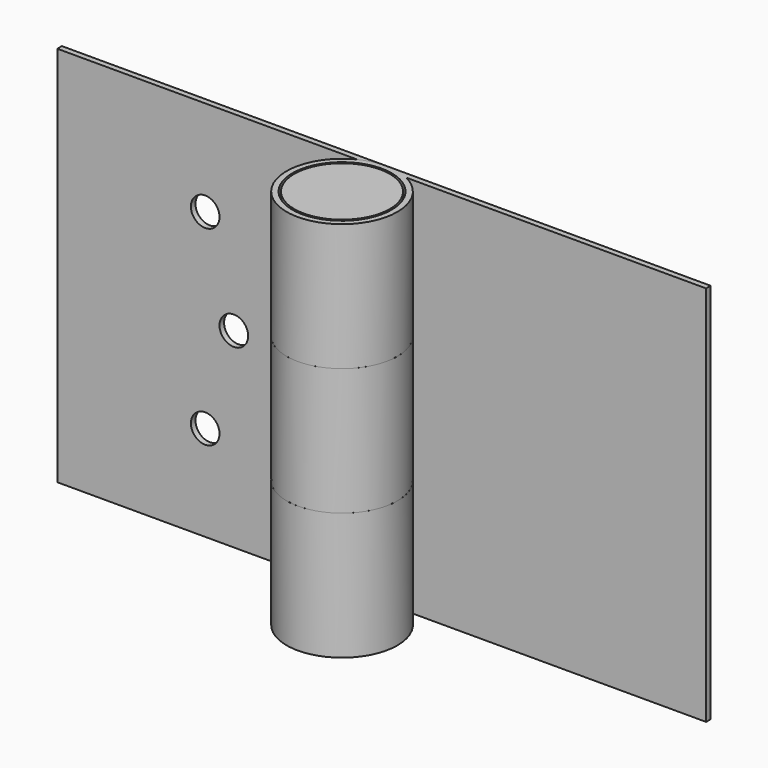
from build123d import *

# Parameters (mm, degrees)
F1_W      = 25
F1_H      = 200
F3_R      = 29
F3_R_2    = 26
F4_DEPTH  = 66.6666666667
F5_START  = -133.332
F5_DEPTH  = 66.668
F6_START  = -66.6666666667
F6_DEPTH  = 66.6666666667
F7_W      = 170
F7_H      = 3
F8_DEPTH  = 200
F9_W      = 170
F9_H      = 3
F10_DEPTH = 200
F11_R     = 7.5
F12_DEPTH = 25


with BuildPart() as f2:
    # F1 (on Front) → F2 (revolve)
    with BuildSketch(Plane.XZ):
        with Locations((-12.5, 0)):
            Rectangle(F1_W, F1_H)
    revolve(axis=Axis((0, 0, 0), (0, 0, -1)))


with BuildPart() as f4:
    # F3 (on face) → F4 (new body)
    with BuildSketch(Plane.XY.offset(100)):
        Circle(F3_R)
        Circle(F3_R_2, mode=Mode.SUBTRACT)
    extrude(amount=-F4_DEPTH)



with BuildPart() as f5:
    # F3 (on face) → F5 (new body)
    with BuildSketch(Plane.XY.offset(100).offset(F5_START)):
        Circle(F3_R)
        Circle(F3_R_2, mode=Mode.SUBTRACT)
    extrude(amount=-F5_DEPTH)


with BuildPart() as f6:
    # F3 (on face) → F6 (new body)
    with BuildSketch(Plane.XY.offset(100).offset(F6_START)):
        Circle(F3_R)
        Circle(F3_R_2, mode=Mode.SUBTRACT)
    extrude(amount=-F6_DEPTH)

    # F9 (on face) → F10 (join)
    with BuildSketch(Plane.XY.offset(100)):
        with Locations((-85, 27.5)):
            Rectangle(F9_W, F9_H)
    extrude(amount=-F10_DEPTH)

    # F11 (on face) → F12 (cut)
    with BuildSketch(Plane(origin=(0, 29, 0), x_dir=(-1, 0, 0), z_dir=(0, 1, 0))):
        with Locations((77.5, 0)):
            Circle(F11_R)
        with Locations((92.5, 50)):
            Circle(F11_R)
        with Locations((92.5, -50)):
            Circle(F11_R)
    extrude(amount=-F12_DEPTH, mode=Mode.SUBTRACT)


with BuildPart() as f4_1:
    add(f4.part)

    add(f5.part)  # F8 merges F5
    # F7 (on face) → F8 (join)
    with BuildSketch(Plane.XY.offset(100)):
        with Locations((85, 27.5)):
            Rectangle(F7_W, F7_H)
    extrude(amount=-F8_DEPTH)


solid = Compound([f2.part, f6.part, f4_1.part])
